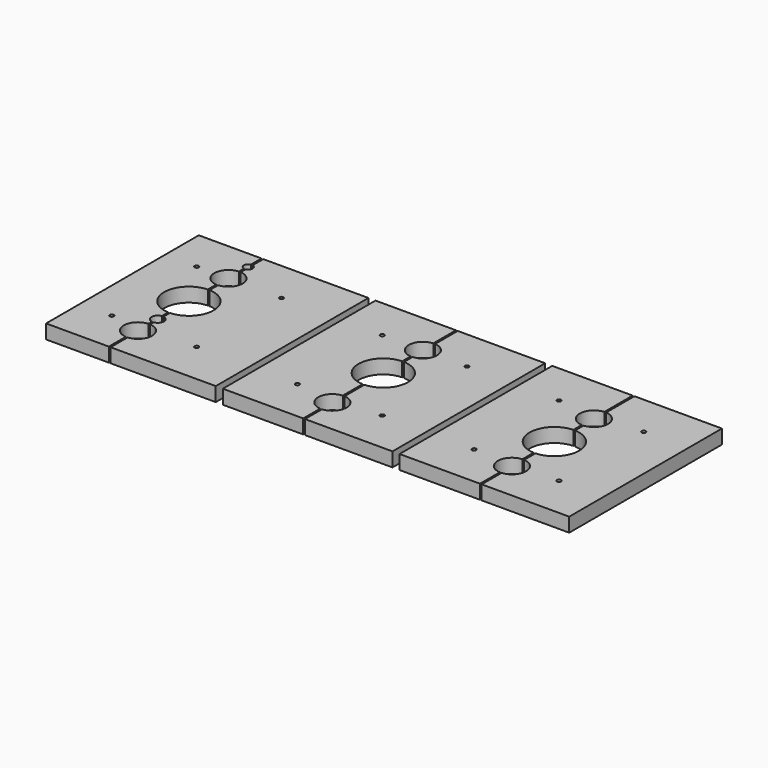
from build123d import *

# Parameters (mm, degrees)
F0_W      = 609.6
F0_H      = 685.8
F1_DEPTH  = 50.8
F2_R      = 50.8
F2_R_2    = 88.9
F2_R_3    = 15.875
F2_R_4    = 22.225
F3_DEPTH  = 50.801
F4_DEPTH  = 635
F10_DEPTH = 685.8
F11_R     = 50.8
F11_R_2   = 88.9
F12_DEPTH = 50.8
F13_DEPTH = 685.8
F14_R     = 50.8
F14_R_2   = 88.9
F15_DEPTH = 50.8
F16_W     = 6.35
F16_H     = 50.8
F17_DEPTH = 685.801
F18_D     = 14.68374
F19_D     = 14.68374
F20_D     = 14.68374


# Not quite as in the source:
# - a feature names something its author has since deleted; it is built from what else it names


with BuildPart() as f1:
    # F0 (on Top) → F1 (new body)
    with BuildSketch(Plane.XY):
        with Locations((304.8, 342.9)):
            Rectangle(F0_W, F0_H)
    extrude(amount=-F1_DEPTH)

    # F2 (on face) → F3 (cut, through all)
    with BuildSketch(Plane.XY):
        with Locations((228.6, 533.4)):
            Circle(F2_R)
        with Locations((228.6, 127)):
            Circle(F2_R)
        with Locations((228.6, 355.6)):
            Circle(F2_R_2)
        with Locations((228.6, 622.3)):
            Circle(F2_R_3)
        with Locations((228.6, 215.9)):
            Circle(F2_R_4)
    extrude(amount=-F3_DEPTH, mode=Mode.SUBTRACT)


with BuildPart() as f4:
    # F4 (new): a face of the model
    f4_faces = [f1.part.faces().sort_by_distance(p)[0] for p in [
        (609.6, 342.9, -25.4),
    ]]
    extrude(f4_faces, amount=F4_DEPTH)


with BuildPart() as f6_1:
    # F6: copy of F1
    add(f1.part)


with BuildPart() as f7_1:
    # F7: copy of F1
    add(f1.part)


with BuildPart() as f6_1_1:
    # F8: moved
    add(f6_1.part.moved(Location((635, 0, 0))))

    # F10 (add, through all): a face of the model
    f10_faces = [f6_1_1.faces().sort_by_distance(p)[0] for p in [
        (939.8, 685.8, -25.4),
    ]]
    extrude(f10_faces, amount=-F10_DEPTH)

    # F11 (on face) → F12 (cut, through all)
    with BuildSketch(Plane.XY):
        with Locations((927.1, 533.4)):
            Circle(F11_R)
        with Locations((927.1, 355.6)):
            Circle(F11_R_2)
        with Locations((927.1, 127)):
            Circle(F11_R)
    extrude(amount=-F12_DEPTH, mode=Mode.SUBTRACT)


with BuildPart() as f7_1_1:
    # F9: moved
    add(f7_1.part.moved(Location((1270, 0, 0))))

    # F13 (add, through all): a face of the model
    f13_faces = [f7_1_1.faces().sort_by_distance(p)[0] for p in [
        (1574.8, 685.8, -25.4),
    ]]
    extrude(f13_faces, amount=-F13_DEPTH)

    # F14 (on face) → F15 (cut, through all)
    with BuildSketch(Plane.XY):
        with Locations((1562.1, 508)):
            Circle(F14_R)
        with Locations((1562.1, 330.2)):
            Circle(F14_R_2)
        with Locations((1562.1, 139.7)):
            Circle(F14_R)
    extrude(amount=-F15_DEPTH, mode=Mode.SUBTRACT)


with BuildPart() as f17_tool:
    # F16 (on face) → F17 (new body, through all)
    with BuildSketch(Plane.XZ):
        with Locations((228.6, -25.4)):
            Rectangle(F16_W, F16_H)
        with Locations((927.1, -25.4)):
            Rectangle(F16_W, F16_H)
        with Locations((1562.1, -25.4)):
            Rectangle(F16_W, F16_H)
    extrude(amount=-F17_DEPTH)


with BuildPart() as f1_1:
    add(f1.part)

    # F17: cut by f17_tool
    add(f17_tool.part, mode=Mode.SUBTRACT)

    # F18 (through all)
    with Locations(Plane.XY):
        with Locations((114.3, 533.4), (114.3, 152.4), (419.1, 533.4), (419.1, 152.4)):
            Hole(F18_D / 2)


with BuildPart() as f6_1_2:
    add(f6_1_1.part)

    # F17: cut by f17_tool
    add(f17_tool.part, mode=Mode.SUBTRACT)

    # F19 (through all)
    with Locations(Plane.XY):
        with Locations((781.05, 533.4), (1085.85, 533.4), (1085.85, 152.4), (781.05, 152.4)):
            Hole(F19_D / 2)


with BuildPart() as f7_1_2:
    add(f7_1_1.part)

    # F17: cut by f17_tool
    add(f17_tool.part, mode=Mode.SUBTRACT)

    # F20 (through all)
    with Locations(Plane.XY):
        with Locations((1416.05, 533.4), (1720.85, 533.4), (1416.05, 152.4), (1720.85, 152.4)):
            Hole(F20_D / 2)


solid = Compound([f1_1.part, f6_1_2.part, f7_1_2.part])
